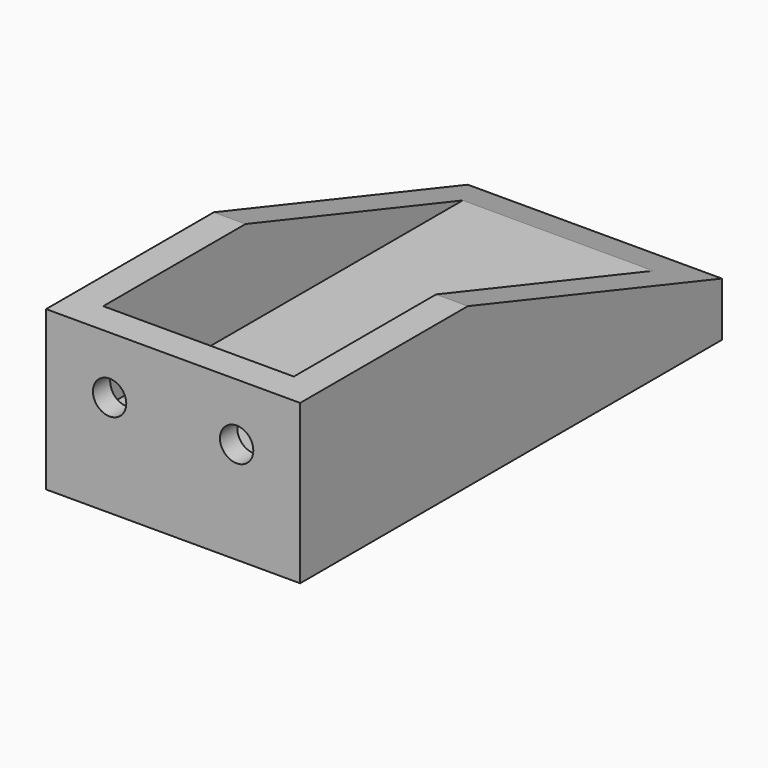
from build123d import *

# Parameters (mm, degrees)
F1_DEPTH       = 40
F3_W           = 30
F3_H           = 28
F3_H_2         = 45
F4_DEPTH       = 14.1
F6_D           = 5.25
F6_DEPTH       = 5
F6_CBORE_D     = 9.75
F6_CBORE_DEPTH = 1.6
F6_TIP         = 1.5772591249
F7_D           = 2.5
F7_DEPTH       = 10
F7_TIP         = 0.7510757738


# Not quite as in the source:
# - a feature names something its author has since deleted; it is built from what else it names


with BuildPart() as f1:
    # F0 (on Right) → F1 (new body)
    with BuildSketch(Plane.YZ):
        Polygon((0, 0), (-78, 0), (-78, 16.5), (-83, 16.5), (-83, -8.5), (0, -8.5), align=None)
        Polygon((-78, 16.5), (-78, 0), (0, 0), (-50, 16.5), align=None)
    extrude(amount=F1_DEPTH)

    # F3 (on face) → F4 (cut)
    with BuildSketch(Plane.XY.offset(16.5)):
        with Locations((20, -64)):
            Rectangle(F3_W, F3_H)
        with Locations((20, -27.5)):
            Rectangle(F3_W, F3_H_2)
    extrude(amount=-F4_DEPTH, mode=Mode.SUBTRACT)

    # F6
    with Locations(Plane(origin=(0, -78, 0), x_dir=(-1, 0, 0), z_dir=(0, 1, 0))):
        with Locations((-30, 7.5), (-10, 7.5)):
            CounterBoreHole(F6_D / 2, F6_CBORE_D / 2, F6_CBORE_DEPTH, depth=F6_DEPTH)
            with Locations((0, 0, -(F6_DEPTH + F6_TIP / 2))):  # 118° drill point
                Cone(0, F6_D / 2, F6_TIP, mode=Mode.SUBTRACT)

    # F7
    with Locations(Plane(origin=(0, 0, -8.5), x_dir=(1, 0, 0), z_dir=(0, 0, -1))):
        with Locations((24, 30), (24, 19), (32, 19), (24, 8)):
            Hole(F7_D / 2, depth=F7_DEPTH)
            with Locations((0, 0, -(F7_DEPTH + F7_TIP / 2))):  # 118° drill point
                Cone(0, F7_D / 2, F7_TIP, mode=Mode.SUBTRACT)


solid = f1.part
